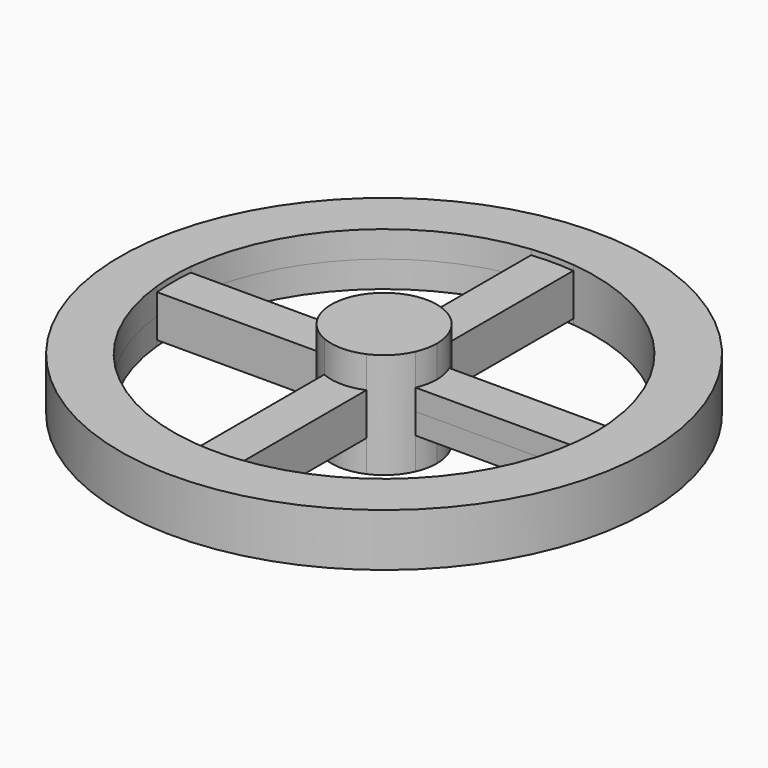
from build123d import *

# Parameters (mm, degrees)
F0_R     = 250
F1_DEPTH = 25
F0_W     = 40
F0_H     = 40
F2_DEPTH = 50
F3_DEPTH = 20


with BuildPart() as f1:
    # F0 (on Top) → F1 (new body, symmetric)
    with BuildSketch(Plane.XY):
        Circle(F0_R)
        with BuildLine():
            ThreePointArc((20, 198.9974874213), (141.4213562373, 141.4213562373), (198.9974874213, 20))
            Line((198.9974874213, 20), (220.8077311516, 20))
            Line((220.8077311516, 20), (220.8077311516, -20))
            Line((220.8077311516, -20), (198.9974874213, -20))
            ThreePointArc((198.9974874213, -20), (141.4213562373, -141.4213562373), (20, -198.9974874213))
            Line((20, -198.9974874213), (20, -220.8077311516))
            Line((20, -220.8077311516), (-20, -220.8077311516))
            Line((-20, -220.8077311516), (-20, -198.9974874213))
            ThreePointArc((-20, -198.9974874213), (-141.4213562373, -141.4213562373), (-198.9974874213, -20))
            Line((-198.9974874213, -20), (-220.8077311516, -20))
            Line((-220.8077311516, -20), (-220.8077311516, 20))
            Line((-220.8077311516, 20), (-198.9974874213, 20))
            ThreePointArc((-198.9974874213, 20), (-141.4213562373, 141.4213562373), (-20, 198.9974874213))
            Line((-20, 198.9974874213), (-20, 220.8077311516))
            Line((-20, 220.8077311516), (20, 220.8077311516))
            Line((20, 220.8077311516), (20, 198.9974874213))
        make_face(mode=Mode.SUBTRACT)
        with BuildLine():
            ThreePointArc((-198.9974874213, -20), (-200, 0), (-198.9974874213, 20))
            Line((-198.9974874213, 20), (-220.8077311516, 20))
            Line((-220.8077311516, 20), (-220.8077311516, -20))
            Line((-220.8077311516, -20), (-198.9974874213, -20))
        make_face()
        with BuildLine():
            Line((20, -220.8077311516), (20, -198.9974874213))
            ThreePointArc((20, -198.9974874213), (0, -200), (-20, -198.9974874213))
            Line((-20, -198.9974874213), (-20, -220.8077311516))
            Line((-20, -220.8077311516), (20, -220.8077311516))
        make_face()
        with BuildLine():
            Line((220.8077311516, 20), (198.9974874213, 20))
            ThreePointArc((198.9974874213, 20), (199.7492146221, 10.012555012), (200, 0))
            ThreePointArc((200, 0), (199.7492146221, -10.012555012), (198.9974874213, -20))
            Line((198.9974874213, -20), (220.8077311516, -20))
            Line((220.8077311516, -20), (220.8077311516, 20))
        make_face()
        with BuildLine():
            ThreePointArc((-20, 198.9974874213), (0, 200), (20, 198.9974874213))
            Line((20, 198.9974874213), (20, 220.8077311516))
            Line((20, 220.8077311516), (-20, 220.8077311516))
            Line((-20, 220.8077311516), (-20, 198.9974874213))
        make_face()
    extrude(amount=F1_DEPTH, both=True)



with BuildPart() as f2:
    # F0 (on Top) → F2 (new body, symmetric)
    with BuildSketch(Plane.XY):
        with BuildLine():
            Line((20, 20), (45.8257569496, 20))
            ThreePointArc((45.8257569496, 20), (35.3553390593, 35.3553390593), (20, 45.8257569496))
            Line((20, 45.8257569496), (20, 20))
        make_face()
        with BuildLine():
            Line((20, 20), (20, 45.8257569496))
            ThreePointArc((20, 45.8257569496), (0, 50), (-20, 45.8257569496))
            Line((-20, 45.8257569496), (-20, 20))
            Line((-20, 20), (20, 20))
        make_face()
        with BuildLine():
            Line((-20, 20), (-20, 45.8257569496))
            ThreePointArc((-20, 45.8257569496), (-35.3553390593, 35.3553390593), (-45.8257569496, 20))
            Line((-45.8257569496, 20), (-20, 20))
        make_face()
        with BuildLine():
            Line((-20, -20), (-20, 20))
            Line((-20, 20), (-45.8257569496, 20))
            ThreePointArc((-45.8257569496, 20), (-50, 0), (-45.8257569496, -20))
            Line((-45.8257569496, -20), (-20, -20))
        make_face()
        with BuildLine():
            ThreePointArc((-45.8257569496, -20), (-35.3553390593, -35.3553390593), (-20, -45.8257569496))
            Line((-20, -45.8257569496), (-20, -20))
            Line((-20, -20), (-45.8257569496, -20))
        make_face()
        with BuildLine():
            ThreePointArc((-20, -45.8257569496), (0, -50), (20, -45.8257569496))
            Line((20, -45.8257569496), (20, -20))
            Line((20, -20), (-20, -20))
            Line((-20, -20), (-20, -45.8257569496))
        make_face()
        with BuildLine():
            ThreePointArc((20, -45.8257569496), (35.3553390593, -35.3553390593), (45.8257569496, -20))
            Line((45.8257569496, -20), (20, -20))
            Line((20, -20), (20, -45.8257569496))
        make_face()
        with BuildLine():
            ThreePointArc((45.8257569496, -20), (48.9453156465, -10.2154821845), (50, 0))
            ThreePointArc((50, 0), (48.9453156465, 10.2154821845), (45.8257569496, 20))
            Line((45.8257569496, 20), (20, 20))
            Line((20, 20), (20, -20))
            Line((20, -20), (45.8257569496, -20))
        make_face()
        with BuildLine():
            Line((-20, -20), (-20, 20))
            Line((-20, 20), (-45.8257569496, 20))
            ThreePointArc((-45.8257569496, 20), (-50, 0), (-45.8257569496, -20))
            Line((-45.8257569496, -20), (-20, -20))
        make_face()
        Rectangle(F0_W, F0_H)
        with BuildLine():
            ThreePointArc((-20, -45.8257569496), (0, -50), (20, -45.8257569496))
            Line((20, -45.8257569496), (20, -20))
            Line((20, -20), (-20, -20))
            Line((-20, -20), (-20, -45.8257569496))
        make_face()
        with BuildLine():
            ThreePointArc((45.8257569496, -20), (48.9453156465, -10.2154821845), (50, 0))
            ThreePointArc((50, 0), (48.9453156465, 10.2154821845), (45.8257569496, 20))
            Line((45.8257569496, 20), (20, 20))
            Line((20, 20), (20, -20))
            Line((20, -20), (45.8257569496, -20))
        make_face()
        with BuildLine():
            Line((20, 20), (20, 45.8257569496))
            ThreePointArc((20, 45.8257569496), (0, 50), (-20, 45.8257569496))
            Line((-20, 45.8257569496), (-20, 20))
            Line((-20, 20), (20, 20))
        make_face()
    extrude(amount=F2_DEPTH, both=True)


with BuildPart() as f1_1:
    add(f1.part)

    add(f2.part)  # F3 merges F2
    # F0 (on Top) → F3 (join, symmetric)
    with BuildSketch(Plane.XY):
        with BuildLine():
            ThreePointArc((-45.8257569496, -20), (-50, 0), (-45.8257569496, 20))
            Line((-45.8257569496, 20), (-198.9974874213, 20))
            ThreePointArc((-198.9974874213, 20), (-200, 0), (-198.9974874213, -20))
            Line((-198.9974874213, -20), (-45.8257569496, -20))
        make_face()
        with BuildLine():
            ThreePointArc((-20, 45.8257569496), (0, 50), (20, 45.8257569496))
            Line((20, 45.8257569496), (20, 198.9974874213))
            ThreePointArc((20, 198.9974874213), (0, 200), (-20, 198.9974874213))
            Line((-20, 198.9974874213), (-20, 45.8257569496))
        make_face()
        with BuildLine():
            ThreePointArc((45.8257569496, 20), (48.9453156465, 10.2154821845), (50, 0))
            ThreePointArc((50, 0), (48.9453156465, -10.2154821845), (45.8257569496, -20))
            Line((45.8257569496, -20), (198.9974874213, -20))
            ThreePointArc((198.9974874213, -20), (199.7492146221, -10.012555012), (200, 0))
            ThreePointArc((200, 0), (199.7492146221, 10.012555012), (198.9974874213, 20))
            Line((198.9974874213, 20), (45.8257569496, 20))
        make_face()
        with BuildLine():
            Line((20, -198.9974874213), (20, -45.8257569496))
            ThreePointArc((20, -45.8257569496), (0, -50), (-20, -45.8257569496))
            Line((-20, -45.8257569496), (-20, -198.9974874213))
            ThreePointArc((-20, -198.9974874213), (0, -200), (20, -198.9974874213))
        make_face()
    extrude(amount=F3_DEPTH, both=True)

    # F4 (on Front) → F5 (revolve, cut)
    with BuildSketch(Plane.XZ):
        Polygon((0, -50), (0, 0), (-24, 0), (-32, -50), align=None)
    revolve(axis=Axis((0, 0, -25), (0, 0, -1)), mode=Mode.SUBTRACT)


solid = f1_1.part
